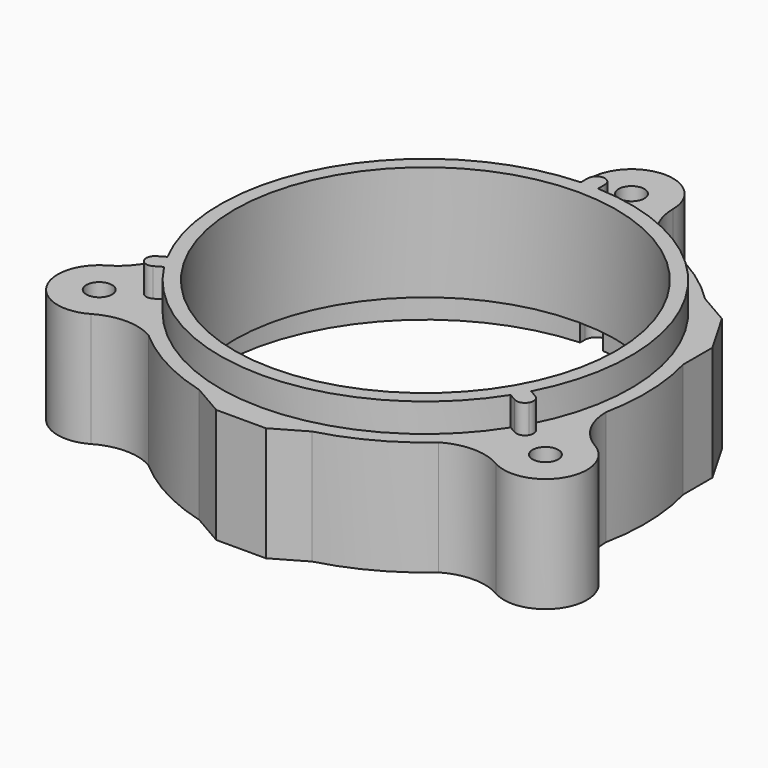
from build123d import *

# Parameters (mm, degrees)
F0_R     = 2.25
F0_R_2   = 33.35
F1_DEPTH = 20
F2_R     = 33.35
F3_DEPTH = 25
F5_DEPTH = 5
F6_R     = 1.49999
F8_DEPTH = 5
F9_SIZE  = 5


# Not quite as in the source:
# - a fillet or chamfer is up to 0.001 mm smaller than in the source, because OpenCascade refuses the exact size


with BuildPart() as f1:
    # F0 (on Top) → F1 (new body)
    with BuildSketch(Plane.XY):
        with BuildLine():
            ThreePointArc((-35.3461431703, -28.7786841774), (-30.3488782685, -27.4389385893), (-25.3508812473, -28.775950375))
            ThreePointArc((-25.3508812473, -28.775950375), (0, -38.35), (25.3508812473, -28.775950375))
            ThreePointArc((25.3508812473, -28.775950375), (30.3488782685, -27.4389385893), (35.3461431703, -28.7786841774))
            ThreePointArc((35.3461431703, -28.7786841774), (45.2498273477, -26.125), (42.5961431703, -16.2213158226))
            ThreePointArc((42.5961431703, -16.2213158226), (38.9372570055, -12.5634302623), (37.5961446665, -7.566531981))
            ThreePointArc((37.5961446665, -7.566531981), (33.2120742351, 19.175), (12.2452634191, 36.342482356))
            ThreePointArc((12.2452634191, 36.342482356), (8.588378737, 40.0023688516), (7.25, 45))
            ThreePointArc((7.25, 45), (0, 52.25), (-7.25, 45))
            ThreePointArc((-7.25, 45), (-8.588378737, 40.0023688516), (-12.2452634191, 36.342482356))
            ThreePointArc((-12.2452634191, 36.342482356), (-33.2120742351, 19.175), (-37.5961446665, -7.566531981))
            ThreePointArc((-37.5961446665, -7.566531981), (-38.9372570055, -12.5634302623), (-42.5961431703, -16.2213158226))
            ThreePointArc((-42.5961431703, -16.2213158226), (-45.2498273477, -26.125), (-35.3461431703, -28.7786841774))
        make_face()
        with Locations((-38.9711431703, -22.5)):
            Circle(F0_R, mode=Mode.SUBTRACT)
        with Locations((38.9711431703, -22.5)):
            Circle(F0_R, mode=Mode.SUBTRACT)
        Circle(F0_R_2, mode=Mode.SUBTRACT)
        with Locations((0, 45)):
            Circle(F0_R, mode=Mode.SUBTRACT)
    extrude(amount=F1_DEPTH)

    # F2 (on Top) → F3 (join)
    with BuildSketch(Plane.XY):
        Polygon((37.0225860118, -21.375), (37.0225860118, 21.375), (0, 42.75), (-37.0225860118, 21.375), (-37.0225860118, -21.375), (0, -42.75), align=None)
        Circle(F2_R, mode=Mode.SUBTRACT)
    extrude(amount=F3_DEPTH)

    # F4 (on face) → F5 (cut)
    with BuildSketch(Plane.XY.offset(25)):
        Polygon((37.0225860118, -21.375), (37.0225860118, 21.375), (0, 42.75), (-37.0225860118, 21.375), (-37.0225860118, -21.375), (0, -42.75), align=None)
        with BuildLine():
            ThreePointArc((-31.7698222916, -16.6102646446), (-31.0470107257, 17.925), (-1.5, 35.8186055005))
            Line((-1.5, 35.8186055005), (-1.5, 38.8186055005))
            Line((-1.5, 38.8186055005), (0, 38.8186055005))
            Line((0, 38.8186055005), (1.5, 38.8186055005))
            Line((1.5, 38.8186055005), (1.5, 35.8186055005))
            ThreePointArc((1.5, 35.8186055005), (31.0470107257, 17.925), (31.7698222916, -16.6102646446))
            Line((31.7698222916, -16.6102646446), (34.3678985029, -18.1102646446))
            Line((34.3678985029, -18.1102646446), (33.6178985029, -19.4093027502))
            Line((33.6178985029, -19.4093027502), (32.8678985029, -20.7083408559))
            Line((32.8678985029, -20.7083408559), (30.2698222916, -19.2083408559))
            ThreePointArc((30.2698222916, -19.2083408559), (0, -35.85), (-30.2698222916, -19.2083408559))
            Line((-30.2698222916, -19.2083408559), (-32.8678985029, -20.7083408559))
            Line((-32.8678985029, -20.7083408559), (-33.6178985029, -19.4093027502))
            Line((-33.6178985029, -19.4093027502), (-34.3678985029, -18.1102646446))
            Line((-34.3678985029, -18.1102646446), (-31.7698222916, -16.6102646446))
        make_face(mode=Mode.SUBTRACT)
    extrude(amount=-F5_DEPTH, mode=Mode.SUBTRACT)

    # F6 (radius 1.5 in the source; OpenCascade refuses exactly that, so slightly less here)
    f6_edges = [f1.edges().sort_by_distance(p)[0] for p in [
        (-32.867899, -20.708341, 22.5),
        (-34.367899, -18.110265, 22.5),
        (32.867899, -20.708341, 22.5),
        (34.367899, -18.110265, 22.5),
        (1.5, 38.818606, 22.5),
        (-1.5, 38.818606, 22.5),
    ]]
    fillet(f6_edges, radius=F6_R)

    # F7 (on Top) → F8 (cut)
    with BuildSketch(Plane.XY):
        with BuildLine():
            Line((-31.3188603972, -20.3913535578), (-30.4323380454, -19.8795196393))
            ThreePointArc((-30.4323380454, -19.8795196393), (0, -36.35), (30.4323380454, -19.8795196393))
            Line((30.4323380454, -19.8795196393), (31.3188603972, -20.3913535578))
            ThreePointArc((31.3188603972, -20.3913535578), (34.0509112048, -19.6593027502), (33.3188603972, -16.9272519427))
            Line((33.3188603972, -16.9272519427), (32.4323380454, -16.4154180242))
            ThreePointArc((32.4323380454, -16.4154180242), (31.4800234276, 18.175), (2, 36.2949376635))
            Line((2, 36.2949376635), (2, 37.3186055005))
            ThreePointArc((2, 37.3186055005), (0, 39.3186055005), (-2, 37.3186055005))
            Line((-2, 37.3186055005), (-2, 36.2949376635))
            ThreePointArc((-2, 36.2949376635), (-31.4800234276, 18.175), (-32.4323380454, -16.4154180242))
            Line((-32.4323380454, -16.4154180242), (-33.3188603972, -16.9272519427))
            ThreePointArc((-33.3188603972, -16.9272519427), (-34.0509112048, -19.6593027502), (-31.3188603972, -20.3913535578))
        make_face()
    extrude(amount=F8_DEPTH, mode=Mode.SUBTRACT)

    # F9
    f9_edges = [f1.edges().sort_by_distance(p)[0] for p in [
        (0, -42.75, 10),
        (37.022586, 21.375, 10),
        (-37.022586, 21.375, 10),
    ]]
    chamfer(f9_edges, length=F9_SIZE)


solid = f1.part
